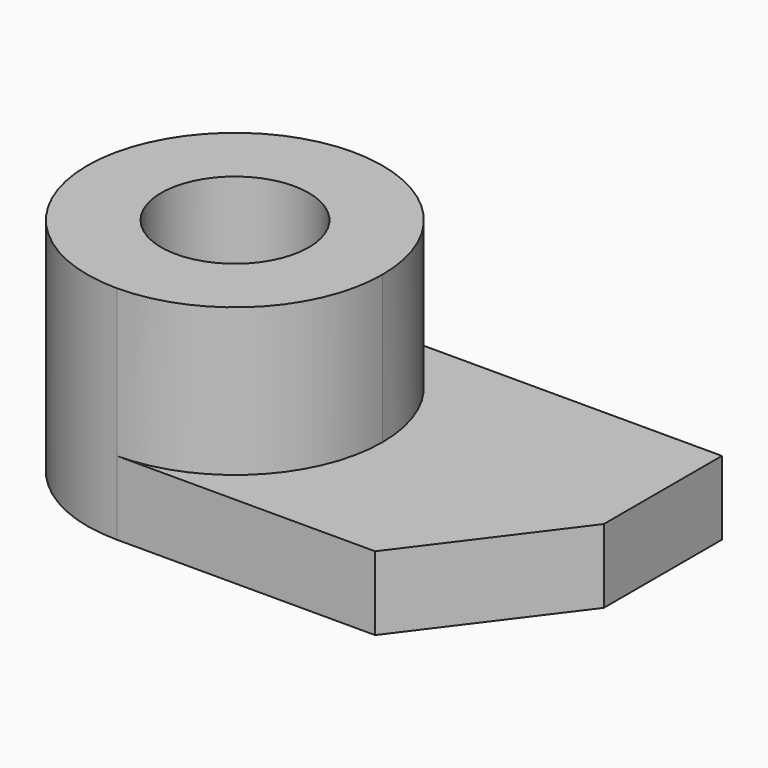
from build123d import *

# Parameters (mm, degrees)
F1_DEPTH = 12.7
F3_DEPTH = 6.351
F4_R     = 6.35
F5_DEPTH = 19.051
F6_R     = 12.7
F7_R     = 12.69999
F8_R     = 12.69999
F9_R     = 12.7


# Not quite as in the source:
# - a fillet or chamfer is up to 0.001 mm smaller than in the source, because OpenCascade refuses the exact size


with BuildPart() as f1:
    # F0 (on Front) → F1 (new body, symmetric)
    with BuildSketch(Plane.XZ):
        Polygon((0, 19.05), (0, 0), (44.45, 0), (44.45, 6.35), (25.4, 6.35), (25.4, 19.05), align=None)
    extrude(amount=F1_DEPTH, both=True)

    # F2 (on face) → F3 (cut, through all)
    with BuildSketch(Plane.XY.offset(6.35)):
        Polygon((34.925, -12.7), (44.45, -12.7), (44.45, 0), align=None)
    extrude(amount=-F3_DEPTH, mode=Mode.SUBTRACT)

    # F4 (on face) → F5 (cut, through all)
    with BuildSketch(Plane.XY.offset(19.05)):
        with Locations((12.7109484747, 0)):
            Circle(F4_R)
    extrude(amount=-F5_DEPTH, mode=Mode.SUBTRACT)

    # F6
    f6_edges = [f1.edges().sort_by_distance(p)[0] for p in [
        (0, -12.7, 9.525),
    ]]
    fillet(f6_edges, radius=F6_R)

    # F7 (radius 12.7 in the source; OpenCascade refuses exactly that, so slightly less here)
    f7_edges = [f1.edges().sort_by_distance(p)[0] for p in [
        (0, 12.7, 9.525),
    ]]
    fillet(f7_edges, radius=F7_R)

    # F8 (radius 12.7 in the source; OpenCascade refuses exactly that, so slightly less here)
    f8_edges = [f1.edges().sort_by_distance(p)[0] for p in [
        (25.4, -12.7, 12.7),
    ]]
    fillet(f8_edges, radius=F8_R)

    # F9
    f9_edges = [f1.edges().sort_by_distance(p)[0] for p in [
        (25.4, 12.7, 12.7),
    ]]
    fillet(f9_edges, radius=F9_R)


solid = f1.part
